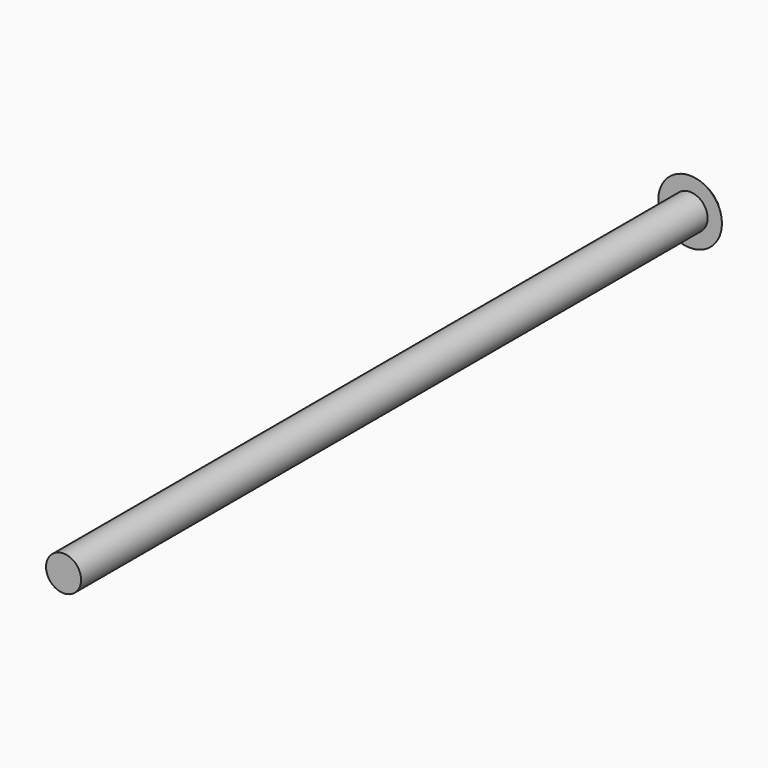
from build123d import *

# Parameters (mm, degrees)
F0_R     = 2.75
F1_DEPTH = 125
F2_R     = 5
F3_DEPTH = 2


# Not quite as in the source:
# - a fillet or chamfer that OpenCascade refuses, or shapes differently, is made with other operations: its cross-section is extruded or revolved along the edge and cut away or added


with BuildPart() as f1:
    # F0 (on Front) → F1 (new body)
    with BuildSketch(Plane.XZ):
        Circle(F0_R)
    extrude(amount=F1_DEPTH)

    # F2 (on Front) → F3 (join)
    with BuildSketch(Plane.XZ):
        Circle(F2_R)
    extrude(amount=F3_DEPTH)

    # F4: fillet of radius 5 on 1 edges, made by hand

    # F4_s1 → F4_t2 (revolve, cut)
    with BuildSketch(Plane.XY):
        with BuildLine():
            ThreePointArc((1, 0), (3.2360679775, -0.527864045), (5, -2))
            Line((5, -2), (5, 0))
            Line((5, 0), (1, 0))
        make_face()
    revolve(axis=Axis((0, 0, 0), (0, -1, 0)), mode=Mode.SUBTRACT)


solid = f1.part
